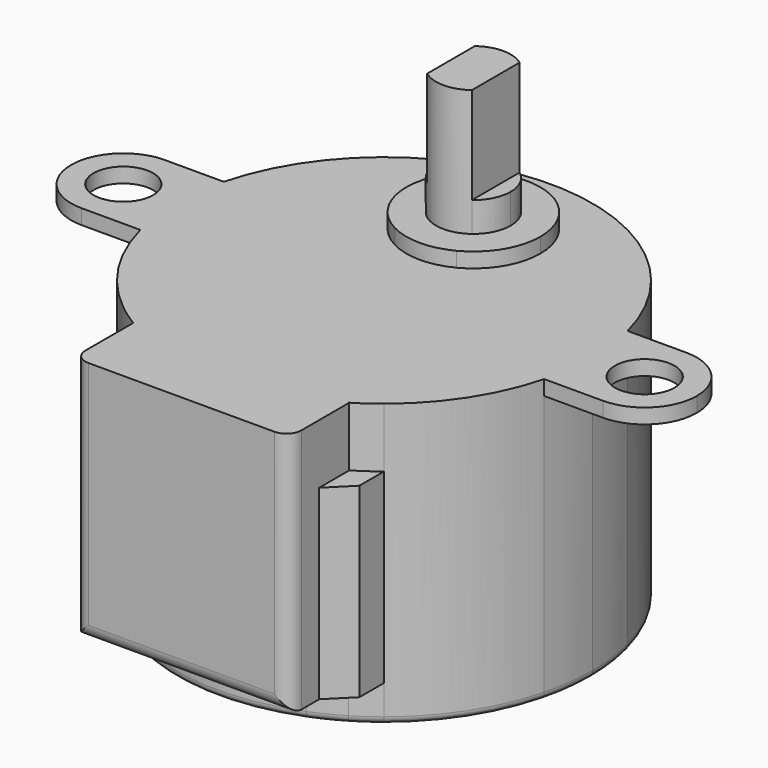
from build123d import *
from build123d import SkipClean  # not in build123d's __all__

# Parameters (mm, degrees)
F0_R          = 2
F1_DEPTH      = 1
F2_DEPTH      = 18
F3_DEPTH      = 15.5
F3_DEPTH_BACK = 1
F4_START      = -3
F4_DEPTH      = 12.5
F5_DEPTH      = 2
F6_DEPTH      = 4
F7_DEPTH      = 10.5
F8_R          = 0.5
F9_R          = 1


with BuildPart() as f1:
    # F0 (on Top) → F1 (new body)
    with BuildSketch(Plane.XY):
        with BuildLine():
            ThreePointArc((2.0615528128, -4), (0, -4.5), (-2.0615528128, -4))
            Line((-2.0615528128, -4), (-13.5554417117, -4))
            ThreePointArc((-13.5554417117, -4), (-13.8884157477, -5.7359399052), (-14, -7.5))
            ThreePointArc((-14, -7.5), (-13.8884157477, -9.2640600948), (-13.5554417117, -11))
            Line((-13.5554417117, -11), (13.5554417117, -11))
            ThreePointArc((13.5554417117, -11), (13.8884157477, -9.2640600948), (14, -7.5))
            ThreePointArc((14, -7.5), (13.8884157477, -5.7359399052), (13.5554417117, -4))
            Line((13.5554417117, -4), (2.0615528128, -4))
        make_face()
        with BuildLine():
            ThreePointArc((17.5, -4), (15.0251262658, -5.0251262658), (14, -7.5))
            ThreePointArc((14, -7.5), (15.0251262658, -9.9748737342), (17.5, -11))
            ThreePointArc((17.5, -11), (19.9748737342, -9.9748737342), (21, -7.5))
            ThreePointArc((21, -7.5), (19.9748737342, -5.0251262658), (17.5, -4))
        make_face()
        with Locations((17.5, -7.5)):
            Circle(F0_R, mode=Mode.SUBTRACT)
        with BuildLine():
            ThreePointArc((-17.5, -11), (-15.0251262658, -9.9748737342), (-14, -7.5))
            ThreePointArc((-14, -7.5), (-15.0251262658, -5.0251262658), (-17.5, -4))
            ThreePointArc((-17.5, -4), (-21, -7.5), (-17.5, -11))
        make_face()
        with Locations((-17.5, -7.5)):
            Circle(F0_R, mode=Mode.SUBTRACT)
        with BuildLine():
            ThreePointArc((-14, -7.5), (-13.8884157477, -5.7359399052), (-13.5554417117, -4))
            Line((-13.5554417117, -4), (-17.5, -4))
            ThreePointArc((-17.5, -4), (-15.0251262658, -5.0251262658), (-14, -7.5))
        make_face()
        with BuildLine():
            ThreePointArc((-13.5554417117, -11), (-13.8884157477, -9.2640600948), (-14, -7.5))
            ThreePointArc((-14, -7.5), (-15.0251262658, -9.9748737342), (-17.5, -11))
            Line((-17.5, -11), (-13.5554417117, -11))
        make_face()
        with BuildLine():
            Line((13.5554417117, -11), (-13.5554417117, -11))
            ThreePointArc((-13.5554417117, -11), (-11.7549883504, -15.1039627091), (-8.75, -18.4287464972))
            Line((-8.75, -18.4287464972), (-8.75, -12.5))
            Line((-8.75, -12.5), (8.75, -12.5))
            Line((8.75, -12.5), (8.75, -18.4287464972))
            ThreePointArc((8.75, -18.4287464972), (11.7549883504, -15.1039627091), (13.5554417117, -11))
        make_face()
        with BuildLine():
            Line((-8.75, -12.5), (-8.75, -18.4287464972))
            ThreePointArc((-8.75, -18.4287464972), (-7.9985057778, -18.9901655916), (-7.2111025509, -19.5))
            Line((-7.2111025509, -19.5), (7.2111025509, -19.5))
            ThreePointArc((7.2111025509, -19.5), (7.9985057778, -18.9901655916), (8.75, -18.4287464972))
            Line((8.75, -18.4287464972), (8.75, -12.5))
            Line((8.75, -12.5), (-8.75, -12.5))
        make_face()
        with BuildLine():
            ThreePointArc((-2.0615528128, -4), (-2.3423292192, 3.8423292192), (4.5, 0))
            ThreePointArc((4.5, 0), (3.8423292192, -2.3423292192), (2.0615528128, -4))
            Line((2.0615528128, -4), (13.5554417117, -4))
            ThreePointArc((13.5554417117, -4), (0, 6.5), (-13.5554417117, -4))
            Line((-13.5554417117, -4), (-2.0615528128, -4))
        make_face()
        with BuildLine():
            Line((17.5, -4), (13.5554417117, -4))
            ThreePointArc((13.5554417117, -4), (13.8884157477, -5.7359399052), (14, -7.5))
            ThreePointArc((14, -7.5), (15.0251262658, -5.0251262658), (17.5, -4))
        make_face()
        with BuildLine():
            ThreePointArc((17.5, -11), (15.0251262658, -9.9748737342), (14, -7.5))
            ThreePointArc((14, -7.5), (13.8884157477, -9.2640600948), (13.5554417117, -11))
            Line((13.5554417117, -11), (17.5, -11))
        make_face()
    extrude(amount=F1_DEPTH)

    # F0 (on Top) → F2 (join)
    with BuildSketch(Plane.XY):
        with BuildLine():
            ThreePointArc((-2.0615528128, -4), (-2.3423292192, 3.8423292192), (4.5, 0))
            ThreePointArc((4.5, 0), (3.8423292192, -2.3423292192), (2.0615528128, -4))
            Line((2.0615528128, -4), (13.5554417117, -4))
            ThreePointArc((13.5554417117, -4), (0, 6.5), (-13.5554417117, -4))
            Line((-13.5554417117, -4), (-2.0615528128, -4))
        make_face()
        with BuildLine():
            ThreePointArc((2.0615528128, -4), (0, -4.5), (-2.0615528128, -4))
            Line((-2.0615528128, -4), (-13.5554417117, -4))
            ThreePointArc((-13.5554417117, -4), (-13.8884157477, -5.7359399052), (-14, -7.5))
            ThreePointArc((-14, -7.5), (-13.8884157477, -9.2640600948), (-13.5554417117, -11))
            Line((-13.5554417117, -11), (13.5554417117, -11))
            ThreePointArc((13.5554417117, -11), (13.8884157477, -9.2640600948), (14, -7.5))
            ThreePointArc((14, -7.5), (13.8884157477, -5.7359399052), (13.5554417117, -4))
            Line((13.5554417117, -4), (2.0615528128, -4))
        make_face()
        with BuildLine():
            Line((13.5554417117, -11), (-13.5554417117, -11))
            ThreePointArc((-13.5554417117, -11), (-11.7549883504, -15.1039627091), (-8.75, -18.4287464972))
            Line((-8.75, -18.4287464972), (-8.75, -12.5))
            Line((-8.75, -12.5), (8.75, -12.5))
            Line((8.75, -12.5), (8.75, -18.4287464972))
            ThreePointArc((8.75, -18.4287464972), (11.7549883504, -15.1039627091), (13.5554417117, -11))
        make_face()
        with BuildLine():
            Line((-8.75, -12.5), (-8.75, -18.4287464972))
            ThreePointArc((-8.75, -18.4287464972), (-7.9985057778, -18.9901655916), (-7.2111025509, -19.5))
            Line((-7.2111025509, -19.5), (7.2111025509, -19.5))
            ThreePointArc((7.2111025509, -19.5), (7.9985057778, -18.9901655916), (8.75, -18.4287464972))
            Line((8.75, -18.4287464972), (8.75, -12.5))
            Line((8.75, -12.5), (-8.75, -12.5))
        make_face()
        with BuildLine():
            Line((5.1961524227, -20.5), (-5.1961524227, -20.5))
            ThreePointArc((-5.1961524227, -20.5), (0, -21.5), (5.1961524227, -20.5))
        make_face()
        with BuildLine():
            Line((7.2111025509, -19.5), (-7.2111025509, -19.5))
            ThreePointArc((-7.2111025509, -19.5), (-6.223744371, -20.0405345183), (-5.1961524227, -20.5))
            Line((-5.1961524227, -20.5), (5.1961524227, -20.5))
            ThreePointArc((5.1961524227, -20.5), (6.223744371, -20.0405345183), (7.2111025509, -19.5))
        make_face()
        with BuildLine():
            ThreePointArc((2.0615528128, -4), (3.8423292192, -2.3423292192), (4.5, 0))
            ThreePointArc((4.5, 0), (-2.3423292192, 3.8423292192), (-2.0615528128, -4))
            Line((-2.0615528128, -4), (2.0615528128, -4))
        make_face()
        with BuildLine():
            ThreePointArc((1.5, 2), (2.2360679775, 1.1180339887), (2.5, 0))
            ThreePointArc((2.5, 0), (2.2360679775, -1.1180339887), (1.5, -2))
            Line((1.5, -2), (1.5, -3.1181974337))
            Line((1.5, -3.1181974337), (-1.5, -3.1181974337))
            Line((-1.5, -3.1181974337), (-1.5, -2))
            ThreePointArc((-1.5, -2), (-2.5, 0), (-1.5, 2))
            Line((-1.5, 2), (-1.5, 2.8818025663))
            Line((-1.5, 2.8818025663), (1.5, 2.8818025663))
            Line((1.5, 2.8818025663), (1.5, 2))
        make_face(mode=Mode.SUBTRACT)
        with BuildLine():
            Line((2.0615528128, -4), (-2.0615528128, -4))
            ThreePointArc((-2.0615528128, -4), (0, -4.5), (2.0615528128, -4))
        make_face()
        with BuildLine():
            ThreePointArc((-1.5, 2), (0, 2.5), (1.5, 2))
            Line((1.5, 2), (1.5, 2.8818025663))
            Line((1.5, 2.8818025663), (-1.5, 2.8818025663))
            Line((-1.5, 2.8818025663), (-1.5, 2))
        make_face()
        with BuildLine():
            Line((1.5, -2), (1.5, 2))
            ThreePointArc((1.5, 2), (0, 2.5), (-1.5, 2))
            Line((-1.5, 2), (-1.5, -2))
            ThreePointArc((-1.5, -2), (0, -2.5), (1.5, -2))
        make_face()
        with BuildLine():
            ThreePointArc((1.5, -2), (2.2360679775, -1.1180339887), (2.5, 0))
            ThreePointArc((2.5, 0), (2.2360679775, 1.1180339887), (1.5, 2))
            Line((1.5, 2), (1.5, -2))
        make_face()
        with BuildLine():
            Line((1.5, -3.1181974337), (1.5, -2))
            ThreePointArc((1.5, -2), (0, -2.5), (-1.5, -2))
            Line((-1.5, -2), (-1.5, -3.1181974337))
            Line((-1.5, -3.1181974337), (1.5, -3.1181974337))
        make_face()
        with BuildLine():
            Line((-1.5, -2), (-1.5, 2))
            ThreePointArc((-1.5, 2), (-2.5, 0), (-1.5, -2))
        make_face()
    with SkipClean():  # cleaning this boolean's faces spoils the solid; the shape is the same uncleaned
        extrude(amount=-F2_DEPTH)

    # F0 (on Top) → F3 (join, two sides)
    with BuildSketch(Plane.XY) as f3_sk:
        with BuildLine():
            ThreePointArc((5.1961524227, -20.5), (0, -21.5), (-5.1961524227, -20.5))
            Line((-5.1961524227, -20.5), (-7.25, -20.5))
            Line((-7.25, -20.5), (-7.25, -22))
            Line((-7.25, -22), (-7.25, -24.5))
            Line((-7.25, -24.5), (7.25, -24.5))
            Line((7.25, -24.5), (7.25, -22))
            Line((7.25, -22), (7.25, -20.5))
            Line((7.25, -20.5), (5.1961524227, -20.5))
        make_face()
        with BuildLine():
            ThreePointArc((-5.1961524227, -20.5), (-6.223744371, -20.0405345183), (-7.2111025509, -19.5))
            Line((-7.2111025509, -19.5), (-7.25, -19.5))
            Line((-7.25, -19.5), (-7.25, -20.5))
            Line((-7.25, -20.5), (-5.1961524227, -20.5))
        make_face()
        with BuildLine():
            Line((5.1961524227, -20.5), (-5.1961524227, -20.5))
            ThreePointArc((-5.1961524227, -20.5), (0, -21.5), (5.1961524227, -20.5))
        make_face()
        with BuildLine():
            Line((7.2111025509, -19.5), (-7.2111025509, -19.5))
            ThreePointArc((-7.2111025509, -19.5), (-6.223744371, -20.0405345183), (-5.1961524227, -20.5))
            Line((-5.1961524227, -20.5), (5.1961524227, -20.5))
            ThreePointArc((5.1961524227, -20.5), (6.223744371, -20.0405345183), (7.2111025509, -19.5))
        make_face()
        with BuildLine():
            Line((7.25, -19.5), (7.2111025509, -19.5))
            ThreePointArc((7.2111025509, -19.5), (6.223744371, -20.0405345183), (5.1961524227, -20.5))
            Line((5.1961524227, -20.5), (7.25, -20.5))
            Line((7.25, -20.5), (7.25, -19.5))
        make_face()
    extrude(amount=-F3_DEPTH)
    extrude(f3_sk.sketch, amount=F3_DEPTH_BACK)

    # F0 (on Top) → F4 (join)
    with BuildSketch(Plane.XY.offset(F4_START)):
        with BuildLine():
            Line((8.75, -20.5), (8.75, -18.4287464972))
            ThreePointArc((8.75, -18.4287464972), (7.9985057778, -18.9901655916), (7.2111025509, -19.5))
            Line((7.2111025509, -19.5), (7.25, -19.5))
            Line((7.25, -19.5), (7.25, -20.5))
            Line((7.25, -20.5), (8.75, -20.5))
        make_face()
        Polygon((7.25, -22), (8.75, -20.5), (7.25, -20.5), align=None)
        with BuildLine():
            ThreePointArc((-7.2111025509, -19.5), (-7.9985057778, -18.9901655916), (-8.75, -18.4287464972))
            Line((-8.75, -18.4287464972), (-8.75, -20.5))
            Line((-8.75, -20.5), (-7.25, -20.5))
            Line((-7.25, -20.5), (-7.25, -19.5))
            Line((-7.25, -19.5), (-7.2111025509, -19.5))
        make_face()
        Polygon((-7.25, -20.5), (-8.75, -20.5), (-7.25, -22), align=None)
    extrude(amount=-F4_DEPTH)

    # F0 (on Top) → F5 (join)
    with BuildSketch(Plane.XY):
        with BuildLine():
            ThreePointArc((2.0615528128, -4), (3.8423292192, -2.3423292192), (4.5, 0))
            ThreePointArc((4.5, 0), (-2.3423292192, 3.8423292192), (-2.0615528128, -4))
            Line((-2.0615528128, -4), (2.0615528128, -4))
        make_face()
        with BuildLine():
            ThreePointArc((1.5, 2), (2.2360679775, 1.1180339887), (2.5, 0))
            ThreePointArc((2.5, 0), (2.2360679775, -1.1180339887), (1.5, -2))
            Line((1.5, -2), (1.5, -3.1181974337))
            Line((1.5, -3.1181974337), (-1.5, -3.1181974337))
            Line((-1.5, -3.1181974337), (-1.5, -2))
            ThreePointArc((-1.5, -2), (-2.5, 0), (-1.5, 2))
            Line((-1.5, 2), (-1.5, 2.8818025663))
            Line((-1.5, 2.8818025663), (1.5, 2.8818025663))
            Line((1.5, 2.8818025663), (1.5, 2))
        make_face(mode=Mode.SUBTRACT)
        with BuildLine():
            ThreePointArc((-1.5, 2), (0, 2.5), (1.5, 2))
            Line((1.5, 2), (1.5, 2.8818025663))
            Line((1.5, 2.8818025663), (-1.5, 2.8818025663))
            Line((-1.5, 2.8818025663), (-1.5, 2))
        make_face()
        with BuildLine():
            Line((1.5, -3.1181974337), (1.5, -2))
            ThreePointArc((1.5, -2), (0, -2.5), (-1.5, -2))
            Line((-1.5, -2), (-1.5, -3.1181974337))
            Line((-1.5, -3.1181974337), (1.5, -3.1181974337))
        make_face()
        with BuildLine():
            Line((2.0615528128, -4), (-2.0615528128, -4))
            ThreePointArc((-2.0615528128, -4), (0, -4.5), (2.0615528128, -4))
        make_face()
    extrude(amount=F5_DEPTH)

    # F0 (on Top) → F6 (join)
    with BuildSketch(Plane.XY):
        with BuildLine():
            ThreePointArc((1.5, -2), (2.2360679775, -1.1180339887), (2.5, 0))
            ThreePointArc((2.5, 0), (2.2360679775, 1.1180339887), (1.5, 2))
            Line((1.5, 2), (1.5, -2))
        make_face()
        with BuildLine():
            Line((1.5, -2), (1.5, 2))
            ThreePointArc((1.5, 2), (0, 2.5), (-1.5, 2))
            Line((-1.5, 2), (-1.5, -2))
            ThreePointArc((-1.5, -2), (0, -2.5), (1.5, -2))
        make_face()
        with BuildLine():
            Line((-1.5, -2), (-1.5, 2))
            ThreePointArc((-1.5, 2), (-2.5, 0), (-1.5, -2))
        make_face()
    extrude(amount=F6_DEPTH)

    # F0 (on Top) → F7 (join)
    with BuildSketch(Plane.XY):
        with BuildLine():
            Line((1.5, -2), (1.5, 2))
            ThreePointArc((1.5, 2), (0, 2.5), (-1.5, 2))
            Line((-1.5, 2), (-1.5, -2))
            ThreePointArc((-1.5, -2), (0, -2.5), (1.5, -2))
        make_face()
    extrude(amount=F7_DEPTH)

    # F8
    f8_edges = [f1.edges().sort_by_distance(p)[0] for p in [
        (7.211103, 4.5, -18),
    ]]
    fillet(f8_edges, radius=F8_R)

    # F9
    f9_edges = [f1.edges().sort_by_distance(p)[0] for p in [
        (-7.25, -24.5, -7.25),
        (0, -24.5, -15.5),
        (7.25, -24.5, -7.25),
    ]]
    fillet(f9_edges, radius=F9_R)


solid = f1.part
